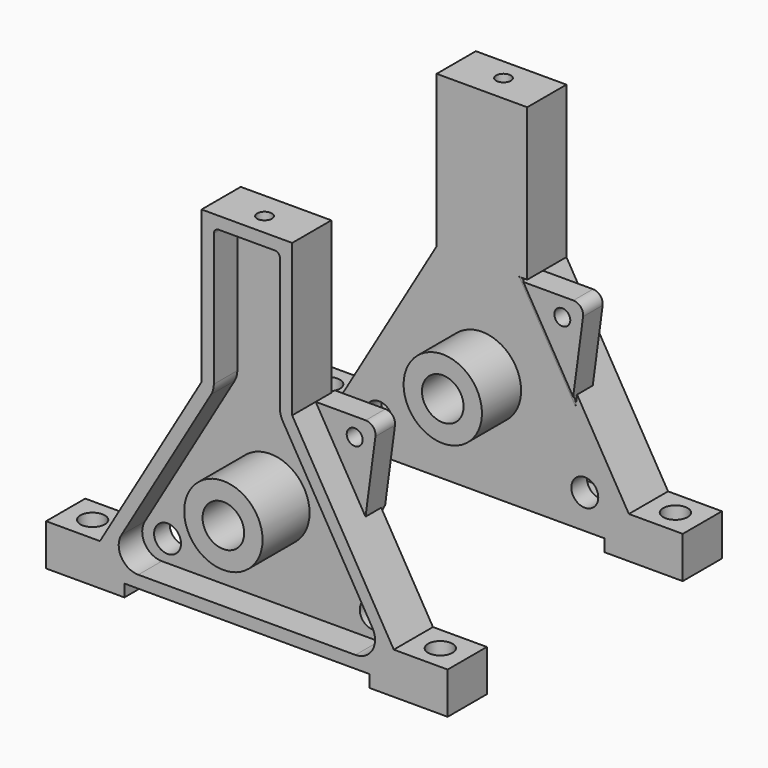
from build123d import *

# Parameters (mm, degrees)
F1_DEPTH       = 20
F4_DEPTH       = 12
F5_R           = 5.5
F6_DEPTH       = 25
F7_R           = 16
F7_R_2         = 8.5
F8_DEPTH       = 24
F9_R           = 16
F9_R_2         = 8.5
F10_DEPTH      = 20
F11_R          = 5
F12_DEPTH      = 25
F13_R          = 3
F14_DEPTH      = 10
F16_R          = 3.25
F17_DEPTH      = 8
F17_DEPTH_BACK = 2
F18_T4_DEPTH   = 54.3641994781


# Not quite as in the source:
# - a fillet or chamfer that OpenCascade refuses, or shapes differently, is made with other operations: its cross-section is extruded or revolved along the edge and cut away or added


with BuildPart() as f1:
    # F0 (on Front) → F1 (new body)
    with BuildSketch(Plane.XZ):
        Polygon((0, 149.7230514048), (-18.5, 149.7230514048), (-18.5, 87.7230514048), (-60, 17), (-82, 17), (-82, 0), (-50, 0), (-50, 5), (0, 5), align=None)
    extrude(amount=F1_DEPTH)

    # F2: F1 across plane


with BuildPart() as f1_1:
    add(f1.part)
    add(f1.part.mirror(Plane.YZ))

    # F3 (on face) → F4 (cut)
    with BuildSketch(Plane.XZ.offset(20)):
        with BuildLine():
            ThreePointArc((44.3403253904, 9.9999997765), (51.2825960529, 14.0244648378), (51.2401352836, 22.0487802643))
            Line((51.2401352836, 22.0487802643), (14.6001903304, 84.489472081))
            ThreePointArc((14.6001903304, 84.489472081), (13.7799458472, 86.4404536205), (13.5000002235, 88.5382525688))
            Line((13.5000002235, 88.5382525688), (13.5000002235, 142.7230516283))
            ThreePointArc((13.5000002235, 142.7230516283), (12.9142137859, 144.1372651906), (11.5000002235, 144.7230516283))
            Line((11.5000002235, 144.7230516283), (-11.5000002235, 144.7230516283))
            ThreePointArc((-11.5000002235, 144.7230516283), (-12.9142137859, 144.1372651906), (-13.5000002235, 142.7230516283))
            Line((-13.5000002235, 142.7230516283), (-13.5000002235, 88.5382525688))
            ThreePointArc((-13.5000002235, 88.5382525688), (-13.7799458472, 86.4404536205), (-14.6001903304, 84.489472081))
            Line((-14.6001903304, 84.489472081), (-51.2401352836, 22.0487802643))
            ThreePointArc((-51.2401352836, 22.0487802643), (-51.2825960529, 14.0244648378), (-44.3403253904, 9.9999997765))
            Line((-44.3403253904, 9.9999997765), (44.3403253904, 9.9999997765))
        make_face()
    extrude(amount=-F4_DEPTH, mode=Mode.SUBTRACT)

    # F5 (on face) → F6 (cut)
    with BuildSketch(Plane.XZ.offset(8)):
        with Locations((-42, 18.8791340478)):
            Circle(F5_R)
        with Locations((42, 18.8791340478)):
            Circle(F5_R)
    extrude(amount=-F6_DEPTH, mode=Mode.SUBTRACT)

    # F7 (on face) → F8 (join)
    with BuildSketch(Plane.XZ.offset(8)):
        with Locations((0, 46.9999997765)):
            Circle(F7_R)
        with Locations((0, 46.9999997765)):
            Circle(F7_R_2, mode=Mode.SUBTRACT)
    extrude(amount=F8_DEPTH)

    # F9 (on face) → F10 (join)
    with BuildSketch(Plane(origin=(0, 0, 0), x_dir=(-1, 0, 0), z_dir=(0, 1, 0))):
        with Locations((0, 46.9999997765)):
            Circle(F9_R)
        with Locations((0, 46.9999997765)):
            Circle(F9_R_2, mode=Mode.SUBTRACT)
    extrude(amount=F10_DEPTH)

    # F11 (on face) → F12 (cut)
    with BuildSketch(Plane.XY.offset(17)):
        with Locations((-71, -10)):
            Circle(F11_R)
        with Locations((71, -10)):
            Circle(F11_R)
    extrude(amount=-F12_DEPTH, mode=Mode.SUBTRACT)

    # F13 (on face) → F14 (cut)
    with BuildSketch(Plane.XY.offset(149.7230514048)):
        with Locations((0, -11)):
            Circle(F13_R)
    extrude(amount=-F14_DEPTH, mode=Mode.SUBTRACT)

    # F16 (on face) → F17 (join, two sides)
    with BuildSketch(Plane(origin=(0, 0, 0), x_dir=(-1, 0, 0), z_dir=(0, 1, 0))) as f17_sk:
        with BuildLine():
            Line((-38.8562884141, 53.0324771416), (-18.5, 87.7230514048))
            Line((-18.5, 87.7230514048), (-38.9288780249, 87.7230514048))
            ThreePointArc((-38.9288780249, 87.7230514048), (-41.9390972513, 86.3571698928), (-42.8935150835, 83.1923415092))
            Line((-42.8935150835, 83.1923415092), (-38.8562884141, 53.0324771416))
        make_face()
        with Locations((-34.4246865011, 80.2230514048)):
            Circle(F16_R, mode=Mode.SUBTRACT)
    extrude(amount=-F17_DEPTH)
    extrude(f17_sk.sketch, amount=F17_DEPTH_BACK)

    # F18: fillet of radius 3 on 1 edges, made by hand


with BuildPart() as f18_tool2:
    # F18_s3 → F18_t4 (new body)
    with BuildSketch(Plane(origin=(-37.1310167355, 0, 63.2775615735), x_dir=(0, 1, 0), z_dir=(0.506097561, 0, -0.8624762366))):
        with BuildLine():
            ThreePointArc((2, 60.3522327352), (0.5505102572, 59.255856418), (0, 57.5238056104))
            Line((0, 57.5238056104), (0, 60.3522327352))
            Line((0, 60.3522327352), (2, 60.3522327352))
        make_face()
    extrude(amount=F18_T4_DEPTH)

    split(bisect_by=Plane(origin=(31.1982792576, 0, -4.176229824), x_dir=(0, 1, 0), z_dir=(-0.9911592647, 0, 0.1326774739)), keep=Keep.TOP)

    split(bisect_by=Plane.XY.offset(87.7230514048), keep=Keep.BOTTOM)


with BuildPart() as f1_2:
    add(f1_1.part)

    # F18_t1: union F18_tool2
    add(f18_tool2.part)


with BuildPart() as f19_1:
    # F19: instance of F1
    add(f1_2.part.mirror(Plane(origin=(0, 50, 55.7488868878), x_dir=(-1, 0, 0), z_dir=(0, 1, 0))))


solid = Compound([f1_2.part, f19_1.part])
